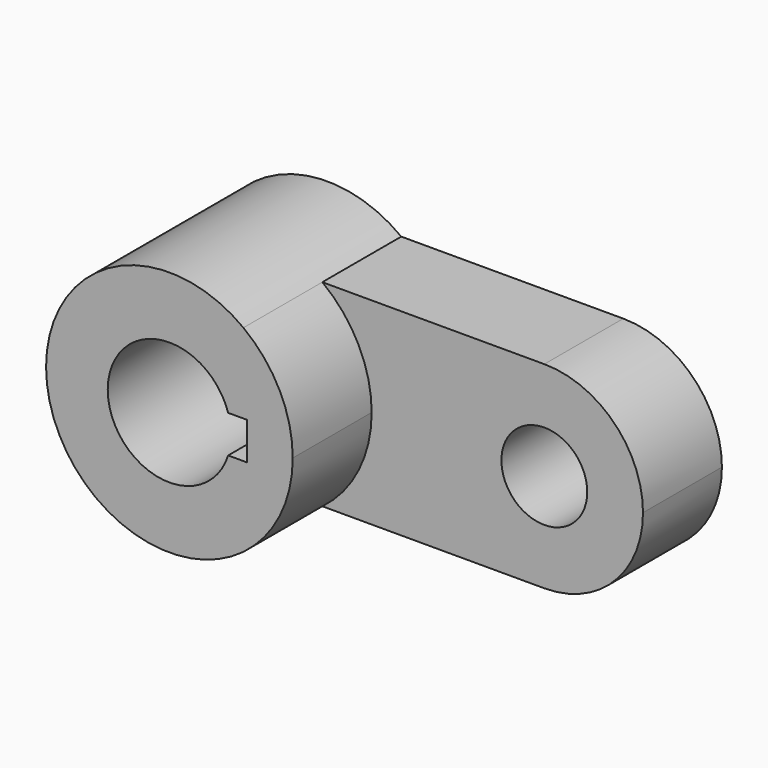
from build123d import *

# Parameters (mm, degrees)
F0_R     = 11.049
F1_DEPTH = 25.4
F2_DEPTH = 50.8


# Not quite as in the source:
# - a feature names something its author has since deleted; it is built from what else it names


with BuildPart() as f1:
    # F0 (on Front) → F1 (new body)
    with BuildSketch(Plane.XZ):
        with BuildLine():
            ThreePointArc((101.6, 0), (94.1605122421, 17.9605122421), (76.2, 25.4))
            ThreePointArc((76.2, 25.4), (50.8, 0), (76.2, -25.4))
            ThreePointArc((76.2, -25.4), (94.1605122421, -17.9605122421), (101.6, 0))
        make_face()
        with Locations((76.2, 0)):
            Circle(F0_R, mode=Mode.SUBTRACT)
        with BuildLine():
            ThreePointArc((19.05, 25.4), (28.3980633142, 14.1990316571), (31.75, 0))
            ThreePointArc((31.75, 0), (28.3980633142, -14.1990316571), (19.05, -25.4))
            Line((19.05, -25.4), (76.2, -25.4))
            ThreePointArc((76.2, -25.4), (50.8, 0), (76.2, 25.4))
            Line((76.2, 25.4), (19.05, 25.4))
        make_face()
    extrude(amount=F1_DEPTH)

    # F0 (on Front) → F2 (join)
    with BuildSketch(Plane.XZ):
        with BuildLine():
            ThreePointArc((19.05, -25.4), (28.3980633142, -14.1990316571), (31.75, 0))
            ThreePointArc((31.75, 0), (28.3980633142, 14.1990316571), (19.05, 25.4))
            ThreePointArc((19.05, 25.4), (-31.75, 0), (19.05, -25.4))
        make_face()
        with BuildLine():
            ThreePointArc((15.1236685034, -4.826), (-15.875, 0), (15.1236685034, 4.826))
            Line((15.1236685034, 4.826), (19.9496685034, 4.826))
            Line((19.9496685034, 4.826), (19.9496685034, -4.826))
            Line((19.9496685034, -4.826), (15.1236685034, -4.826))
        make_face(mode=Mode.SUBTRACT)
    extrude(amount=F2_DEPTH)


solid = f1.part
